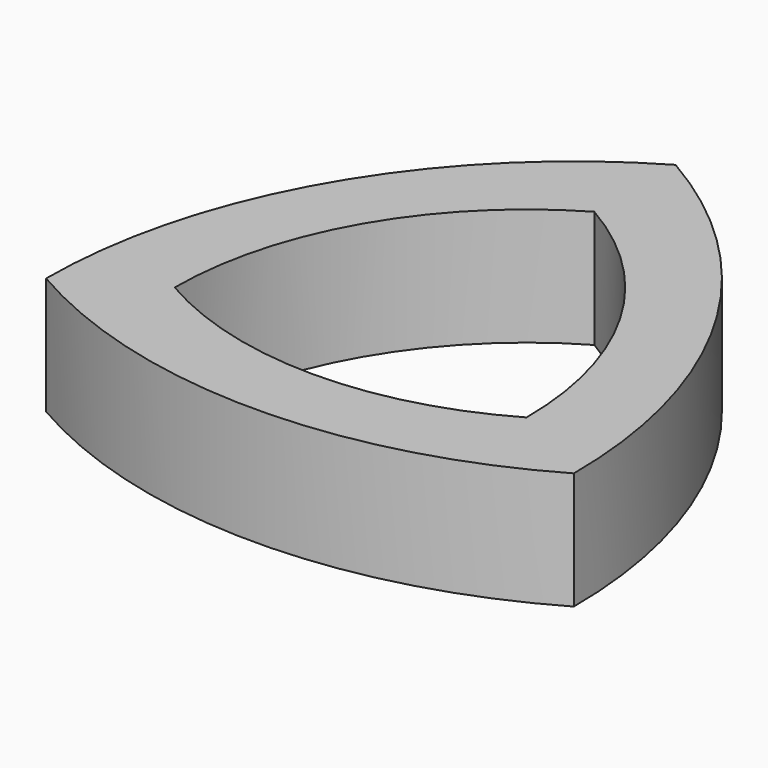
from build123d import *

# Parameters (mm, degrees)
F2_DEPTH = 6.35
F3_DEPTH = 6.35


# Not quite as in the source:
# - a feature of the source that left no trace in its solid (it failed there, or was rolled back) is left out


with BuildPart() as f2:
    # F1 (on Top) → F2 (new body)
    with BuildSketch(Plane.XY):
        with BuildLine():
            ThreePointArc((14.2875, -8.248891971), (10.4591759131, 6.038608029), (0, 16.4977839421))
            ThreePointArc((0, 16.4977839421), (-10.4591759131, 6.038608029), (-14.2875, -8.248891971))
            ThreePointArc((-14.2875, -8.248891971), (0, -12.0772160579), (14.2875, -8.248891971))
        make_face()
    extrude(amount=F2_DEPTH)

    # F0 (on Top) → F3 (cut, through all)
    with BuildSketch(Plane.XY):
        with BuildLine():
            ThreePointArc((9.525, -5.499261314), (6.9727839421, 4.025738686), (0, 10.9985226281))
            ThreePointArc((0, 10.9985226281), (-6.9727839421, 4.025738686), (-9.525, -5.499261314))
            ThreePointArc((-9.525, -5.499261314), (0, -8.0514773719), (9.525, -5.499261314))
        make_face()
    extrude(amount=F3_DEPTH, mode=Mode.SUBTRACT)


solid = f2.part
